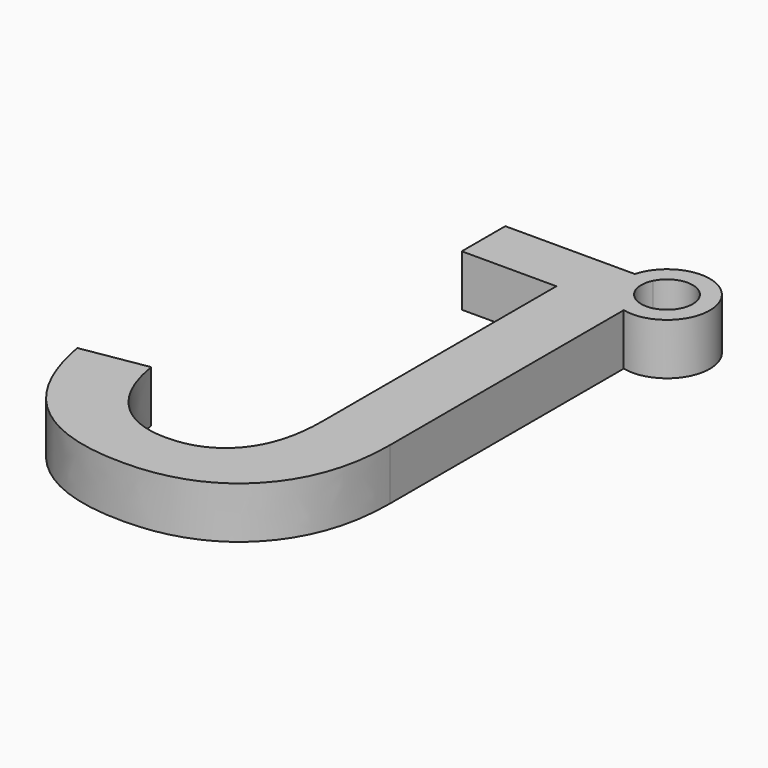
from build123d import *

# Parameters (mm, degrees)
F1_DEPTH = 3


with BuildPart() as f1:
    # F0 (on Top) → F1 (new body)
    with BuildSketch(Plane.XY):
        with BuildLine():
            ThreePointArc((-50.6740901919, 5.7108190317), (-48.9880719662, 6.5060249327), (-47.8297353387, 5.0454544483))
            ThreePointArc((-47.8297353387, 5.0454544483), (-48.4967601552, 3.7979960948), (-49.9046051304, 3.6599853138))
            Line((-49.9046051304, 3.6599853138), (-49.9046051304, 2.6124471071))
            ThreePointArc((-49.9046051304, 2.6124471071), (-47.7784736714, 3.084947565), (-46.8297353387, 5.0454544483))
            ThreePointArc((-46.8297353387, 5.0454544483), (-48.9940121238, 7.5228098776), (-51.7395672771, 5.7108190317))
            Line((-51.7395672771, 5.7108190317), (-50.6740901919, 5.7108190317))
        make_face()
        with BuildLine():
            ThreePointArc((-49.9046051304, 3.6599853138), (-50.7341339801, 4.518515689), (-50.6740901919, 5.7108190317))
            Line((-50.6740901919, 5.7108190317), (-51.7395672771, 5.7108190317))
            ThreePointArc((-51.7395672771, 5.7108190317), (-51.4808021089, 3.7715189123), (-49.9046051304, 2.6124471071))
            Line((-49.9046051304, 2.6124471071), (-49.9046051304, 3.6599853138))
        make_face()
        with BuildLine():
            ThreePointArc((-49.9046051304, 2.6124471071), (-51.4808021089, 3.7715189123), (-51.7395672771, 5.7108190317))
            Line((-51.7395672771, 5.7108190317), (-59.286115547, 5.7108190317))
            Line((-59.286115547, 5.7108190317), (-59.286115547, 2.540246115))
            Line((-59.286115547, 2.540246115), (-53.7717926304, 2.540246115))
            Line((-53.7717926304, 2.540246115), (-53.7717926304, -14.491003885))
            add(Edge.make_bspline(
                [(-54.9924957554, -18.7520715933), (-53.7717926304, -17.2969934683), (-53.7717926304, -14.491003885)],
                knots=[0, 0, 0, 1, 1, 1], degree=2))
            add(Edge.make_bspline(
                [(-58.329084297, -20.2071497183), (-56.2131988804, -20.2071497183), (-54.9924957554, -18.7520715933)],
                knots=[0, 0, 0, 1, 1, 1], degree=2))
            add(Edge.make_bspline(
                [(-61.541974922, -18.885535135), (-60.262678047, -20.2071497183), (-58.329084297, -20.2071497183)],
                knots=[0, 0, 0, 1, 1, 1], degree=2))
            add(Edge.make_bspline(
                [(-63.192365547, -15.2006393017), (-62.821271797, -17.5639205517), (-61.541974922, -18.885535135)],
                knots=[0, 0, 0, 1, 1, 1], degree=2))
            Line((-63.192365547, -15.2006393017), (-66.9944488804, -15.8321497183))
            add(Edge.make_bspline(
                [(-58.348615547, -23.3647018017), (-65.633771797, -23.3647018017), (-66.9944488804, -15.8321497183)],
                knots=[0, 0, 0, 1, 1, 1], degree=2))
            add(Edge.make_bspline(
                [(-52.1637197137, -20.9721236767), (-54.422834297, -23.3647018017), (-58.348615547, -23.3647018017)],
                knots=[0, 0, 0, 1, 1, 1], degree=2))
            add(Edge.make_bspline(
                [(-49.9046051304, -14.4063684683), (-49.9046051304, -18.5795455517), (-52.1637197137, -20.9721236767)],
                knots=[0, 0, 0, 1, 1, 1], degree=2))
            Line((-49.9046051304, -14.4063684683), (-49.9046051304, 2.6124471071))
        make_face()
    extrude(amount=F1_DEPTH)


solid = f1.part
